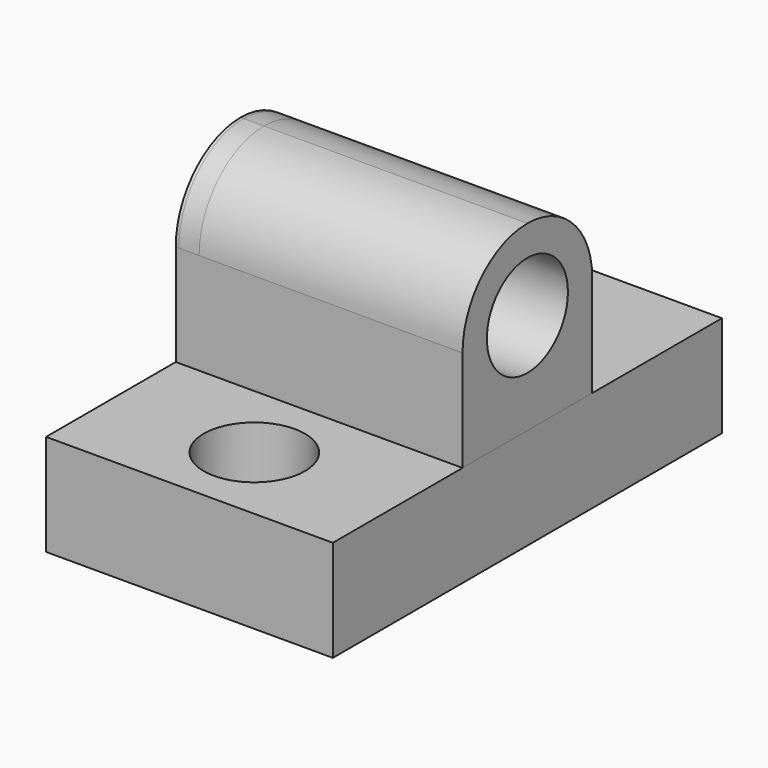
from build123d import *

# Parameters (mm, degrees)
F0_W      = 179.7395497561
F0_H      = 101.6
F0_R      = 31.75
F1_DEPTH  = 25.4
F1_FACE_W = 179.7395497561
F1_FACE_H = 304.8
F1_FACE_R = 31.75
F2_DEPTH  = 38.1
F3_W      = 179.7395497561
F3_H      = 101.6
F4_DEPTH  = 114.3
F5_R      = 31.75
F6_DEPTH  = 177.8
F7_R      = 31.75
F8_DEPTH  = 12.7


with BuildPart() as f1:
    # F0 (on Top) → F1 (new body)
    with BuildSketch(Plane.XY):
        with Locations((46.2416782975, 0)):
            Rectangle(F0_W, F0_H)
        with Locations((46.2416782975, 0)):
            Circle(F0_R, mode=Mode.SUBTRACT)
        with Locations((46.2416782975, -101.6)):
            Rectangle(F0_W, F0_H)
        with Locations((46.2416782975, -203.2)):
            Rectangle(F0_W, F0_H)
        with Locations((46.2416782975, -203.2)):
            Circle(F0_R, mode=Mode.SUBTRACT)
    extrude(amount=F1_DEPTH)

    # F0 (on Top) + F1_face (on face) → F2 (join)
    with BuildSketch(Plane.XY):
        with Locations((46.2416782975, 0)):
            Rectangle(F0_W, F0_H)
        with Locations((46.2416782975, 0)):
            Circle(F0_R, mode=Mode.SUBTRACT)
        with Locations((46.2416782975, -101.6)):
            Rectangle(F0_W, F0_H)
        with Locations((46.2416782975, -203.2)):
            Rectangle(F0_W, F0_H)
        with Locations((46.2416782975, -203.2)):
            Circle(F0_R, mode=Mode.SUBTRACT)
    with BuildSketch(Plane(origin=(46.2416782975, -101.6, 25.4), x_dir=(1, 0, 0), z_dir=(0, 0, 1))):
        Rectangle(F1_FACE_W, F1_FACE_H)
        with Locations((0, 101.6)):
            Circle(F1_FACE_R, mode=Mode.SUBTRACT)
        with Locations((0, -101.6)):
            Circle(F1_FACE_R, mode=Mode.SUBTRACT)
    extrude(amount=F2_DEPTH)


with BuildPart() as f4:
    # F3 (on face) → F4 (new body)
    with BuildSketch(Plane.XY.offset(63.5)):
        with Locations((46.2416782975, -101.6)):
            Rectangle(F3_W, F3_H)
    extrude(amount=F4_DEPTH)

    # F5 (on face) → F6 (cut, symmetric)
    with BuildSketch(Plane.YZ.offset(136.1114531755)):
        with Locations((-101.6, 127)):
            Circle(F5_R)
        with BuildLine():
            ThreePointArc((-152.4, 127), (-137.5210244843, 162.9210244843), (-101.6, 177.8))
            Line((-101.6, 177.8), (-152.4, 177.8))
            Line((-152.4, 177.8), (-152.4, 127))
        make_face()
        with BuildLine():
            ThreePointArc((-101.6, 177.8), (-65.6789755157, 162.9210244843), (-50.8, 127))
            Line((-50.8, 127), (-50.8, 160.3168845177))
            Line((-50.8, 160.3168845177), (-50.8, 177.8))
            Line((-50.8, 177.8), (-101.6, 177.8))
        make_face()
    extrude(amount=F6_DEPTH, both=True, mode=Mode.SUBTRACT)

    # F6_face (on face) + F7 (on face) → F8 (cut, symmetric)
    with BuildSketch(Plane(origin=(-41.6885468245, -101.6, 127), x_dir=(0, 1, 0), z_dir=(1, 0, 0))):
        with BuildLine():
            ThreePointArc((-50.8, 0), (-35.9210244843, 35.9210244843), (0, 50.8))
            Line((0, 50.8), (-50.8, 50.8))
            Line((-50.8, 50.8), (-50.8, 0))
        make_face()
        with BuildLine():
            Line((50.8, 50.8), (0, 50.8))
            ThreePointArc((0, 50.8), (35.9210244843, 35.9210244843), (50.8, 0))
            Line((50.8, 0), (50.8, 50.8))
        make_face()
    with BuildSketch(Plane.YZ.offset(-41.6885468245)):
        with Locations((-101.6, 127)):
            Circle(F7_R)
    extrude(amount=F8_DEPTH, both=True, mode=Mode.SUBTRACT)


solid = Compound([f1.part, f4.part])
